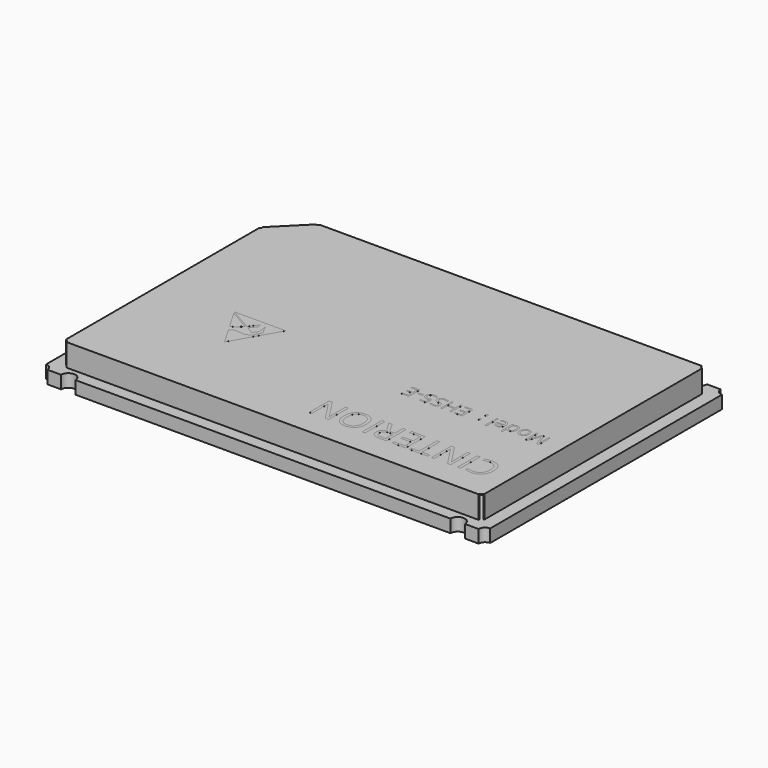
from build123d import *

# Parameters (mm, degrees)
F1_DEPTH        = 1.4
F2_DEPTH        = 0.8
F3_T            = -0.05
F4_R            = 0.45
F4_R_2          = 0.1
F5_DEPTH        = 2
F6_W            = 0.8
F6_H            = 1.5
F6_W_2          = 1.1
F6_H_2          = 1.1
F6_H_3          = 0.55
F6_W_3          = 1.5
F6_H_4          = 0.8
F7_DEPTH        = 0.05
F8_DEPTH        = 0.03
F9_DEPTH        = 0.03
F10_TEXT_SIZE   = 2.1466351528
F10_TEXT_SIZE_2 = 1.2051281778
F11_DEPTH       = 0.001


# Not quite as in the source:
# - Text() gives the source's letters only with a copy of the font that has no kerning and outlines rounded to 1/6400 em; it was checked with that copy


with BuildPart() as f1:
    # F0 (on Top) → F1 (new body)
    with BuildSketch(Plane.XY):
        Polygon((-13, -8.65), (13, -8.65), (13, 8.65), (-11, 8.65), (-13, 6.65), align=None)
    extrude(amount=F1_DEPTH)

    # F3
    f3_openings = [f1.faces().sort_by_distance(p)[0] for p in [
        (0.055084, -0.035656, 0),
    ]]
    offset(amount=F3_T, openings=f3_openings)

    # F4 (on face) → F5 (cut)
    with BuildSketch(Plane.XY.offset(1.4)):
        with Locations((13.2, -8.85)):
            Circle(F4_R)
        with Locations((-13.2, -8.85)):
            Circle(F4_R)
        with Locations((-13, 6.65)):
            Circle(F4_R_2)
        with Locations((-11, 8.65)):
            Circle(F4_R_2)
        with Locations((13.2, 8.85)):
            Circle(F4_R)
    extrude(amount=-F5_DEPTH, mode=Mode.SUBTRACT)


with BuildPart() as f2:
    # F0 (on Top) → F2 (new body)
    with BuildSketch(Plane.XY):
        with BuildLine():
            Line((-13.4, -9.4), (-13, -9.4))
            Line((-13, -9.4), (-12.55, -9.4))
            ThreePointArc((-12.55, -9.4), (-12.1, -8.95), (-11.65, -9.4))
            Line((-11.65, -9.4), (11.65, -9.4))
            ThreePointArc((11.65, -9.4), (12.1, -8.95), (12.55, -9.4))
            Line((12.55, -9.4), (13.4, -9.4))
            ThreePointArc((13.4, -9.4), (13.5171572875, -9.1171572875), (13.8, -9))
            Line((13.8, -9), (13.8, 9))
            ThreePointArc((13.8, 9), (13.5171572875, 9.1171572875), (13.4, 9.4))
            Line((13.4, 9.4), (12.55, 9.4))
            ThreePointArc((12.55, 9.4), (12.1, 8.95), (11.65, 9.4))
            Line((11.65, 9.4), (-11.65, 9.4))
            ThreePointArc((-11.65, 9.4), (-12.1, 8.95), (-12.55, 9.4))
            Line((-12.55, 9.4), (-13.4, 9.4))
            ThreePointArc((-13.4, 9.4), (-13.5171572875, 9.1171572875), (-13.8, 9))
            Line((-13.8, 9), (-13.8, -9))
            ThreePointArc((-13.8, -9), (-13.5171572875, -9.1171572875), (-13.4, -9.4))
        make_face()
        Polygon((13, 8.65), (13, -8.65), (-13, -8.65), (-13, 6.65), (-13, 8.65), (-11, 8.65), align=None, mode=Mode.SUBTRACT)
        Polygon((-13, -8.65), (13, -8.65), (13, 8.65), (-11, 8.65), (-13, 6.65), align=None)
        Polygon((-13, 8.65), (-13, 6.65), (-11, 8.65), align=None)
    extrude(amount=-F2_DEPTH)

    # F6 (on face) → F7 (cut)
    with BuildSketch(Plane(origin=(0, 0, -0.8), x_dir=(1, 0, 0), z_dir=(0, 0, -1))):
        with Locations((0, 8.35)):
            Rectangle(F6_W, F6_H)
        with Locations((0, -8.35)):
            Rectangle(F6_W, F6_H)
        with Locations((-1.2, 8.35)):
            Rectangle(F6_W, F6_H)
        with Locations((-1.2, -8.35)):
            Rectangle(F6_W, F6_H)
        with Locations((-2.4, 8.35)):
            Rectangle(F6_W, F6_H)
        with Locations((-2.4, -8.35)):
            Rectangle(F6_W, F6_H)
        with Locations((-3.6, 8.35)):
            Rectangle(F6_W, F6_H)
        with Locations((-3.6, -8.35)):
            Rectangle(F6_W, F6_H)
        with Locations((-4.8, 8.35)):
            Rectangle(F6_W, F6_H)
        with Locations((-4.8, -8.35)):
            Rectangle(F6_W, F6_H)
        with Locations((-6, 8.35)):
            Rectangle(F6_W, F6_H)
        with Locations((-6, -8.35)):
            Rectangle(F6_W, F6_H)
        with Locations((-7.2, 8.35)):
            Rectangle(F6_W, F6_H)
        with Locations((-7.2, -8.35)):
            Rectangle(F6_W, F6_H)
        with Locations((-8.4, 8.35)):
            Rectangle(F6_W, F6_H)
        with Locations((-8.4, -8.35)):
            Rectangle(F6_W, F6_H)
        with Locations((-9.6, 8.35)):
            Rectangle(F6_W, F6_H)
        with Locations((-9.6, -8.35)):
            Rectangle(F6_W, F6_H)
        with Locations((-10.8, 8.35)):
            Rectangle(F6_W, F6_H)
        with Locations((-10.8, -8.35)):
            Rectangle(F6_W, F6_H)
        with Locations((1.2, 8.35)):
            Rectangle(F6_W, F6_H)
        with Locations((1.2, -8.35)):
            Rectangle(F6_W, F6_H)
        with Locations((2.4, 8.35)):
            Rectangle(F6_W, F6_H)
        with Locations((2.4, -8.35)):
            Rectangle(F6_W, F6_H)
        with Locations((3.6, 8.35)):
            Rectangle(F6_W, F6_H)
        with Locations((3.6, -8.35)):
            Rectangle(F6_W, F6_H)
        with Locations((4.8, 8.35)):
            Rectangle(F6_W, F6_H)
        with Locations((4.8, -8.35)):
            Rectangle(F6_W, F6_H)
        with Locations((6, 8.35)):
            Rectangle(F6_W, F6_H)
        with Locations((6, -8.35)):
            Rectangle(F6_W, F6_H)
        with Locations((7.2, 8.35)):
            Rectangle(F6_W, F6_H)
        with Locations((7.2, -8.35)):
            Rectangle(F6_W, F6_H)
        with Locations((8.4, 8.35)):
            Rectangle(F6_W, F6_H)
        with Locations((8.4, -8.35)):
            Rectangle(F6_W, F6_H)
        with Locations((9.6, 8.35)):
            Rectangle(F6_W, F6_H)
        with Locations((9.6, -8.35)):
            Rectangle(F6_W, F6_H)
        with Locations((10.8, 8.35)):
            Rectangle(F6_W, F6_H)
        with Locations((10.8, -8.35)):
            Rectangle(F6_W, F6_H)
        with Locations((0, -6)):
            Rectangle(F6_W_2, F6_H_2)
        with Locations((0, -4)):
            Rectangle(F6_W_2, F6_H_2)
        with Locations((0, 4)):
            Rectangle(F6_W_2, F6_H_2)
        with Locations((0, 6)):
            Rectangle(F6_W_2, F6_H_2)
        with Locations((2, 6)):
            Rectangle(F6_W_2, F6_H_2)
        with Locations((2, 4)):
            Rectangle(F6_W_2, F6_H_2)
        with Locations((2, -6)):
            Rectangle(F6_W_2, F6_H_2)
        with Locations((2, -4)):
            Rectangle(F6_W_2, F6_H_2)
        with Locations((4, 6)):
            Rectangle(F6_W_2, F6_H_2)
        with Locations((4, 4)):
            Rectangle(F6_W_2, F6_H_2)
        with Locations((4, -6)):
            Rectangle(F6_W_2, F6_H_2)
        with Locations((4, -4)):
            Rectangle(F6_W_2, F6_H_2)
        with Locations((6, 6)):
            Rectangle(F6_W_2, F6_H_2)
        with Locations((6, 4)):
            Rectangle(F6_W_2, F6_H_2)
        with Locations((6, -6)):
            Rectangle(F6_W_2, F6_H_2)
        with Locations((6, -4)):
            Rectangle(F6_W_2, F6_H_2)
        with Locations((-2, -4)):
            Rectangle(F6_W_2, F6_H_2)
        with Locations((-2, -6)):
            Rectangle(F6_W_2, F6_H_2)
        with Locations((-2, 6)):
            Rectangle(F6_W_2, F6_H_2)
        with Locations((-2, 4)):
            Rectangle(F6_W_2, F6_H_2)
        with Locations((-4, -4)):
            Rectangle(F6_W_2, F6_H_2)
        with Locations((-4, -6)):
            Rectangle(F6_W_2, F6_H_2)
        with Locations((-4, 6)):
            Rectangle(F6_W_2, F6_H_2)
        with Locations((-4, 4)):
            Rectangle(F6_W_2, F6_H_2)
        with Locations((-6, -4)):
            Rectangle(F6_W_2, F6_H_2)
        with Locations((-6, -6)):
            Rectangle(F6_W_2, F6_H_2)
        with Locations((-6, 6)):
            Rectangle(F6_W_2, F6_H_2)
        with Locations((-6, 4)):
            Rectangle(F6_W_2, F6_H_2)
        with Locations((-8, -0.275)):
            Rectangle(F6_W_2, F6_H_3)
        Polygon((-12, -0.35), (-12.75, -0.35), (-13.5, -0.35), (-13.5, -1.15), (-12, -1.15), align=None)
        Polygon((-13.5, 0.2), (-12.75, 0.2), (-12, 0.2), (-12, 1), (-13.5, 1), align=None)
        with Locations((-10, -0.275)):
            Rectangle(F6_W_2, F6_H_3)
        with Locations((-10, 0.275)):
            Rectangle(F6_W_2, F6_H_3)
        with Locations((-8, 0.275)):
            Rectangle(F6_W_2, F6_H_3)
        with Locations((8, 0)):
            Rectangle(F6_W_2, F6_H_2)
        with Locations((10, 0)):
            Rectangle(F6_W_2, F6_H_2)
        with Locations((-10, 2)):
            Rectangle(F6_W_2, F6_H_2)
        with Locations((-8, 2)):
            Rectangle(F6_W_2, F6_H_2)
        with Locations((8, 2)):
            Rectangle(F6_W_2, F6_H_2)
        with Locations((10, 2)):
            Rectangle(F6_W_2, F6_H_2)
        with Locations((-10, -2)):
            Rectangle(F6_W_2, F6_H_2)
        with Locations((-8, -2)):
            Rectangle(F6_W_2, F6_H_2)
        with Locations((8, -2)):
            Rectangle(F6_W_2, F6_H_2)
        with Locations((10, -2)):
            Rectangle(F6_W_2, F6_H_2)
        with Locations((12.75, 7.8)):
            Rectangle(F6_W_3, F6_H_4)
        with Locations((12.75, 6.6)):
            Rectangle(F6_W_3, F6_H_4)
        with Locations((12.75, 5.4)):
            Rectangle(F6_W_3, F6_H_4)
        with Locations((12.75, 4.2)):
            Rectangle(F6_W_3, F6_H_4)
        with Locations((12.75, 3)):
            Rectangle(F6_W_3, F6_H_4)
        with Locations((12.75, 1.8)):
            Rectangle(F6_W_3, F6_H_4)
        with Locations((12.75, 0.6)):
            Rectangle(F6_W_3, F6_H_4)
        with Locations((12.75, -0.6)):
            Rectangle(F6_W_3, F6_H_4)
        with Locations((12.75, -1.8)):
            Rectangle(F6_W_3, F6_H_4)
        with Locations((12.75, -3)):
            Rectangle(F6_W_3, F6_H_4)
        with Locations((12.75, -4.2)):
            Rectangle(F6_W_3, F6_H_4)
        with Locations((12.75, -5.4)):
            Rectangle(F6_W_3, F6_H_4)
        with Locations((12.75, -6.6)):
            Rectangle(F6_W_3, F6_H_4)
        with Locations((12.75, -7.8)):
            Rectangle(F6_W_3, F6_H_4)
        with Locations((-12.75, 1.95)):
            Rectangle(F6_W_3, F6_H_4)
        with Locations((-12.75, 3.15)):
            Rectangle(F6_W_3, F6_H_4)
        with Locations((-12.75, 4.35)):
            Rectangle(F6_W_3, F6_H_4)
        with Locations((-12.75, 5.55)):
            Rectangle(F6_W_3, F6_H_4)
        with Locations((-12.75, 6.75)):
            Rectangle(F6_W_3, F6_H_4)
        with Locations((-12.75, 7.95)):
            Rectangle(F6_W_3, F6_H_4)
        with Locations((-12.75, -1.95)):
            Rectangle(F6_W_3, F6_H_4)
        with Locations((-12.75, -3.15)):
            Rectangle(F6_W_3, F6_H_4)
        with Locations((-12.75, -4.35)):
            Rectangle(F6_W_3, F6_H_4)
        with Locations((-12.75, -5.55)):
            Rectangle(F6_W_3, F6_H_4)
        with Locations((-12.75, -6.75)):
            Rectangle(F6_W_3, F6_H_4)
        with Locations((-12.75, -7.95)):
            Rectangle(F6_W_3, F6_H_4)
    extrude(amount=-F7_DEPTH, mode=Mode.SUBTRACT)


with BuildPart() as f8:
    # F8 (new): faces of the model
    f8_faces = [f2.part.faces().sort_by_distance(p)[0] for p in [
        (-12.75, -7.95, -0.75),
        (-12.75, -6.75, -0.75),
        (-12.75, -5.55, -0.75),
        (-12.75, -4.35, -0.75),
        (-12.75, -3.15, -0.75),
        (-12.75, -1.95, -0.75),
        (-12.75, -0.6, -0.75),
        (-12.75, 0.75, -0.75),
        (-12.75, 1.95, -0.75),
        (-12.75, 3.15, -0.75),
        (-12.75, 4.35, -0.75),
        (-12.75, 5.55, -0.75),
        (-12.75, 6.75, -0.75),
        (-12.75, 7.95, -0.75),
        (-10.8, 8.35, -0.75),
        (-9.6, 8.35, -0.75),
        (-8.4, 8.35, -0.75),
        (-7.2, 8.35, -0.75),
        (-6, 8.35, -0.75),
        (-4.8, 8.35, -0.75),
        (-10, 2, -0.75),
        (-10, 0, -0.75),
        (-10, -2, -0.75),
        (-8, -2, -0.75),
        (-8, 0, -0.75),
        (-8, 2, -0.75),
        (-6, 4, -0.75),
        (-4, 4, -0.75),
        (-2, 4, -0.75),
        (0, 4, -0.75),
        (2, 4, -0.75),
        (4, 4, -0.75),
        (6, 4, -0.75),
        (6, 6, -0.75),
        (4, 6, -0.75),
        (2, 6, -0.75),
        (0, 6, -0.75),
        (-2, 6, -0.75),
        (-4, 6, -0.75),
        (-6, 6, -0.75),
        (-3.6, 8.35, -0.75),
        (-2.4, 8.35, -0.75),
        (-1.2, 8.35, -0.75),
        (0, 8.35, -0.75),
        (1.2, 8.35, -0.75),
        (2.4, 8.35, -0.75),
        (3.6, 8.35, -0.75),
        (4.8, 8.35, -0.75),
        (6, 8.35, -0.75),
        (7.2, 8.35, -0.75),
        (8.4, 8.35, -0.75),
        (9.6, 8.35, -0.75),
        (10.8, 8.35, -0.75),
        (12.75, 7.8, -0.75),
        (12.75, 6.6, -0.75),
        (12.75, 5.4, -0.75),
        (12.75, 4.2, -0.75),
        (12.75, 3, -0.75),
        (10, 2, -0.75),
        (8, 2, -0.75),
        (8, 0, -0.75),
        (8, -2, -0.75),
        (10, -2, -0.75),
        (10, 0, -0.75),
        (12.75, 1.8, -0.75),
        (12.75, 0.6, -0.75),
        (12.75, -0.6, -0.75),
        (12.75, -1.8, -0.75),
        (12.75, -3, -0.75),
        (-6, -4, -0.75),
        (-6, -6, -0.75),
        (-4, -6, -0.75),
        (-4, -4, -0.75),
        (-2, -6, -0.75),
        (0, -6, -0.75),
        (0, -4, -0.75),
        (2, -4, -0.75),
        (2, -6, -0.75),
        (4, -6, -0.75),
        (4, -4, -0.75),
        (6, -4, -0.75),
        (6, -6, -0.75),
        (12.75, -4.2, -0.75),
        (12.75, -5.4, -0.75),
        (12.75, -6.6, -0.75),
        (12.75, -7.8, -0.75),
        (10.8, -8.35, -0.75),
        (9.6, -8.35, -0.75),
        (8.4, -8.35, -0.75),
        (7.2, -8.35, -0.75),
        (6, -8.35, -0.75),
        (4.8, -8.35, -0.75),
        (3.6, -8.35, -0.75),
        (2.4, -8.35, -0.75),
        (1.2, -8.35, -0.75),
        (0, -8.35, -0.75),
        (-1.2, -8.35, -0.75),
        (-2.4, -8.35, -0.75),
        (-3.6, -8.35, -0.75),
        (-4.8, -8.35, -0.75),
        (-6, -8.35, -0.75),
        (-7.2, -8.35, -0.75),
        (-8.4, -8.35, -0.75),
        (-9.6, -8.35, -0.75),
        (-10.8, -8.35, -0.75),
        (-2, -4, -0.75),
    ]]
    extrude(f8_faces, amount=F8_DEPTH)


with BuildPart() as f9:
    # F9 (new): a face of the model
    f9_faces = [f2.part.faces().sort_by_distance(p)[0] for p in [
        (2, 4, -0.75),
    ]]
    extrude(f9_faces, amount=F9_DEPTH)


with BuildPart() as f11:
    # F10 (on face) → F11 (new body)
    with BuildSketch(Plane.XY.offset(1.4)):
        with BuildLine():
            Line((-6.0328837693, -2.4702560061), (-5.2328837693, -1.08461536))
            Line((-5.2328837693, -1.08461536), (-8.4328837693, -1.08461536))
            Line((-8.4328837693, -1.08461536), (-6.9960047412, -1.9141978537))
            Line((-6.9960047412, -1.9141978537), (-6.5812640823, -1.3517102925))
            Line((-6.5812640823, -1.3517102925), (-6.5328949131, -1.5935538104))
            Line((-6.5328949131, -1.5935538104), (-6.868786398, -1.9876473984))
            Line((-6.868786398, -1.9876473984), (-6.4315300868, -2.2400974473))
            add(Edge.make_bspline(
                [(-6.2991129234, -1.3517102925), (-6.2375623183, -1.5793013683), (-6.1297936228, -1.977789625), (-6.3409659317, -2.1613675319), (-6.4315300868, -2.2400974473)],
                knots=[0, 0, 0, 0, 0.571136218, 1, 1, 1, 1], degree=3))
            Line((-6.2991129234, -1.3517102925), (-5.9683145029, -1.9539860885))
            Line((-5.9683145029, -1.9539860885), (-6.2080082514, -2.3691478392))
            Line((-6.2080082514, -2.3691478392), (-6.0328837693, -2.4702560061))
        make_face()
        with BuildLine():
            Line((-6.0700482801, -2.5346268271), (-6.2551436995, -2.4277619369))
            add(Edge.make_bspline(
                [(-6.2551436995, -2.4277619369), (-6.3408655094, -2.5053778019), (-6.528088036, -2.6748963685), (-7.0295762084, -2.5707424293), (-7.2808443832, -2.580595015), (-7.4033229543, -2.7013303263), (-7.4645988372, -2.7617340586)],
                knots=[0, 0, 0, 0, 0.2588844733, 0.5654220928, 0.7825811916, 1, 1, 1, 1], degree=3))
            Line((-7.4645988372, -2.7617340586), (-6.8328837693, -3.8558966521))
            Line((-6.8328837693, -3.8558966521), (-6.0700482801, -2.5346268271))
        make_face()
        with BuildLine():
            add(Edge.make_bspline(
                [(-7.0440755314, -1.9722719314), (-7.2649877377, -2.1699791804), (-7.5680622007, -2.4412182366), (-7.6644642378, -2.3854183806), (-7.6905984388, -2.3702912661)],
                knots=[0, 0, 0, 0, 0.728904059, 1, 1, 1, 1], degree=3))
            Line((-7.0440755314, -1.9722719314), (-8.3585547476, -1.2133570021))
            Line((-8.3585547476, -1.2133570021), (-7.6905984388, -2.3702912661))
        make_face()
        with Locations(Location((11.964119777, -5.5315382779), (0, 0, -180))):
            Text('CINTERION', F10_TEXT_SIZE, font='Open Sans', text_align=(TextAlign.LEFT, TextAlign.BOTTOM))
        with Locations(Location((11.9416896339, -1.8709613942), (0, 0, -180))):
            Text('Model :  EHS5-E', F10_TEXT_SIZE_2, font='Open Sans', text_align=(TextAlign.LEFT, TextAlign.BOTTOM))
    extrude(amount=F11_DEPTH)


solid = Compound([f1.part, f2.part, f8.part, f9.part, f11.part])
